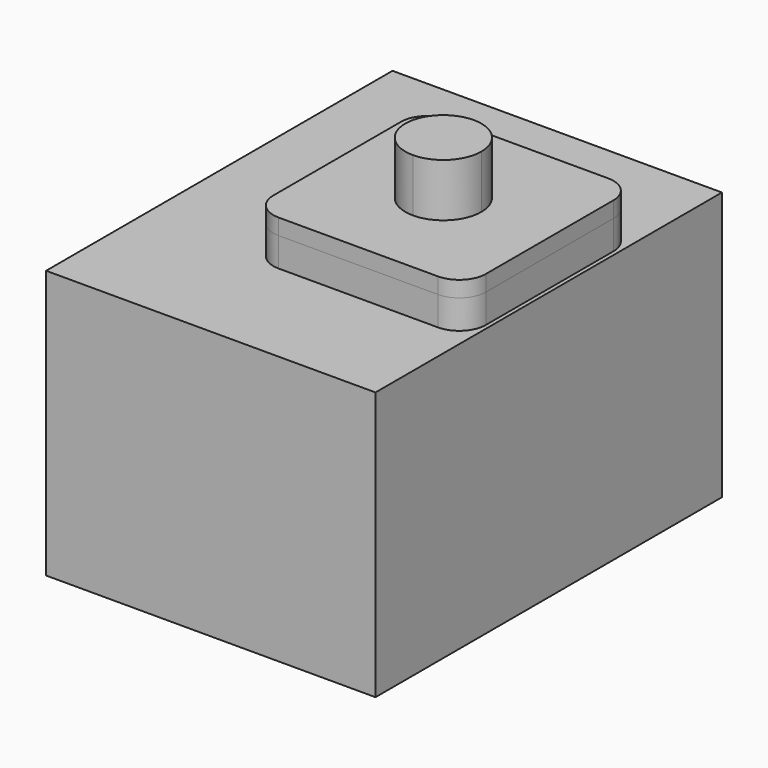
from build123d import *

# Parameters (mm, degrees)
F0_W     = 62
F0_H     = 81.5
F1_DEPTH = 50.5
F2_W     = 40
F2_H     = 40
F3_DEPTH = 5.45
F4_R     = 5
F5_DEPTH = 3
F7_DEPTH = 10


# Not quite as in the source:
# - a feature of the source that left no trace in its solid (it failed there, or was rolled back) is left out


with BuildPart() as f1:
    # F0 (on Top) → F1 (new body)
    with BuildSketch(Plane.XY):
        Rectangle(F0_W, F0_H)
    extrude(amount=F1_DEPTH)

    # F2 (on face) → F3 (join)
    with BuildSketch(Plane.XY.offset(50.5)):
        with Locations((10.25, 1.15)):
            Rectangle(F2_W, F2_H)
    extrude(amount=F3_DEPTH)

    # F4
    f4_edges = [f1.edges().sort_by_distance(p)[0] for p in [
        (-9.75, 21.15, 53.225),
        (-9.75, -18.85, 53.225),
        (30.25, -18.85, 53.225),
        (30.25, 21.15, 53.225),
    ]]
    fillet(f4_edges, radius=F4_R)


with BuildPart() as f5:
    # F5 (new): a face of the model
    f5_faces = [f1.part.faces().sort_by_distance(p)[0] for p in [
        (10.25, 1.15, 55.95),
    ]]
    extrude(f5_faces, amount=F5_DEPTH)

    # F6 (on face) → F7 (join)
    with BuildSketch(Plane.XY.offset(58.95)):
        with BuildLine():
            ThreePointArc((17.4, 1.15), (15.3058134855, 6.2058134855), (10.25, 8.3))
            Line((10.25, 8.3), (10.25, -6))
            ThreePointArc((10.25, -6), (15.3058134855, -3.9058134855), (17.4, 1.15))
        make_face()
        with BuildLine():
            Line((10.25, -6), (10.25, 8.3))
            ThreePointArc((10.25, 8.3), (3.1, 1.15), (10.25, -6))
        make_face()
    extrude(amount=F7_DEPTH)


solid = Compound([f1.part, f5.part])
